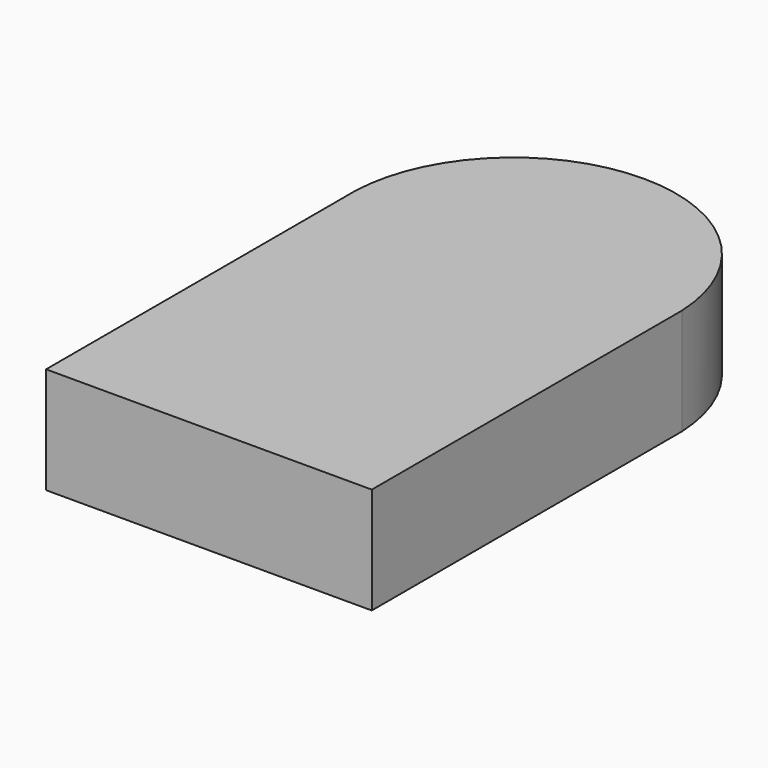
from build123d import *

# Parameters (mm, degrees)
F0_W     = 77.7348391712
F0_H     = 92.5234109163
F1_DEPTH = 25.4


# Not quite as in the source:
# - the program builds the solid bodies; features that only make, move or delete a surface that nothing else refers to are left out


with BuildPart() as f1:
    # F0 (on Top) → F1 (new body)
    with BuildSketch(Plane.XY):
        with BuildLine():
            ThreePointArc((39.2466150224, 36.4026539028), (0.3791954368, 73.5593266262), (-38.4882241488, 36.4026539028))
            Line((-38.4882241488, 36.4026539028), (39.2466150224, 36.4026539028))
        make_face()
        with Locations((0.3791954368, -9.8590515554)):
            Rectangle(F0_W, F0_H)
    extrude(amount=F1_DEPTH)


solid = f1.part
